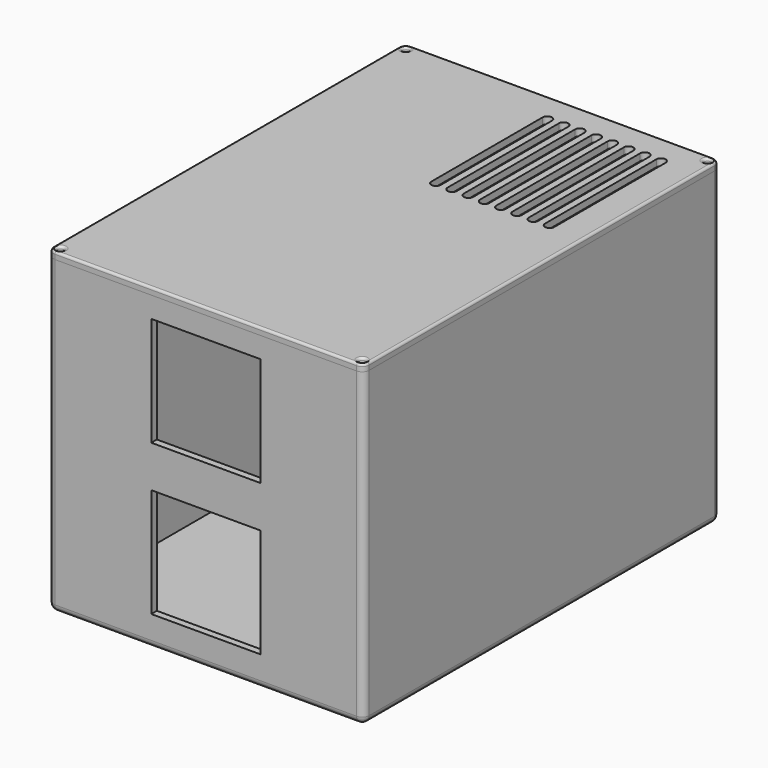
from build123d import *

# Parameters (mm, degrees)
F0_W          = 136
F0_H          = 192
F1_DEPTH      = 4
F2_DEPTH      = 134
F3_W          = 47
F3_H          = 47
F4_DEPTH      = 25
F5_W          = 84
F5_H          = 10
F6_DEPTH      = 20
F8_DEPTH      = 10
F9_W          = 10
F9_H          = 107
F10_DEPTH     = 10
F11_R         = 1.5
F12_DEPTH     = 10
F13_W         = 10
F13_H         = 10
F13_W_2       = 27
F13_H_2       = 68
F13_H_3       = 66
F13_H_4       = 19
F13_R         = 1.6
F14_DEPTH     = 25
F15_R         = 3
F16_R         = 3
F17_R         = 3
F19_W         = 67
F19_H         = 127
F19_W_2       = 47
F19_H_2       = 47
F20_DEPTH     = 10
F21_SIZE      = 1
F23_R         = 1.5
F24_DEPTH     = 3
F25_T1_DEPTH  = 186
F25_T3_DEPTH  = 130
F25_T6_ANGLE  = 90
F25_T8_ANGLE  = 90
F25_T10_ANGLE = 90
F25_T12_ANGLE = 90
F27_DEPTH     = 25
F28_W         = 2.2
F28_H         = 59
F28_H_2       = 5
F29_DEPTH     = 97


# Not quite as in the source:
# - a fillet or chamfer that OpenCascade refuses, or shapes differently, is made with other operations: its cross-section is extruded or revolved along the edge and cut away or added


with BuildPart() as f1:
    # F0 (on Top) → F1 (new body)
    with BuildSketch(Plane.XY):
        Rectangle(F0_W, F0_H)
        with BuildLine():
            ThreePointArc((65, -88), (61.4644660941, -89.4644660941), (60, -93))
            Line((60, -93), (-60, -93))
            ThreePointArc((-60, -93), (-61.4644660941, -89.4644660941), (-65, -88))
            Line((-65, -88), (-65, 88))
            ThreePointArc((-65, 88), (-61.4644660941, 89.4644660941), (-60, 93))
            Line((-60, 93), (60, 93))
            ThreePointArc((60, 93), (61.4644660941, 89.4644660941), (65, 88))
            Line((65, 88), (65, -88))
        make_face(mode=Mode.SUBTRACT)
        with BuildLine():
            Line((-60, -93), (60, -93))
            ThreePointArc((60, -93), (61.4644660941, -89.4644660941), (65, -88))
            Line((65, -88), (65, 88))
            ThreePointArc((65, 88), (61.4644660941, 89.4644660941), (60, 93))
            Line((60, 93), (-60, 93))
            ThreePointArc((-60, 93), (-61.4644660941, 89.4644660941), (-65, 88))
            Line((-65, 88), (-65, -88))
            ThreePointArc((-65, -88), (-61.4644660941, -89.4644660941), (-60, -93))
        make_face()
    extrude(amount=F1_DEPTH)

    # F0 (on Top) → F2 (join)
    with BuildSketch(Plane.XY):
        Rectangle(F0_W, F0_H)
        with BuildLine():
            ThreePointArc((65, -88), (61.4644660941, -89.4644660941), (60, -93))
            Line((60, -93), (-60, -93))
            ThreePointArc((-60, -93), (-61.4644660941, -89.4644660941), (-65, -88))
            Line((-65, -88), (-65, 88))
            ThreePointArc((-65, 88), (-61.4644660941, 89.4644660941), (-60, 93))
            Line((-60, 93), (60, 93))
            ThreePointArc((60, 93), (61.4644660941, 89.4644660941), (65, 88))
            Line((65, 88), (65, -88))
        make_face(mode=Mode.SUBTRACT)
    extrude(amount=F2_DEPTH)

    # F3 (on face) → F4 (cut)
    with BuildSketch(Plane.XZ.offset(96)):
        with Locations((0, 101.5)):
            Rectangle(F3_W, F3_H)
        with Locations((0, 36.5)):
            Rectangle(F3_W, F3_H)
    extrude(amount=-F4_DEPTH, mode=Mode.SUBTRACT)

    # F5 (on face) → F6 (join)
    with BuildSketch(Plane.XY.offset(4)):
        with Locations((-23, 78)):
            Rectangle(F5_W, F5_H)
    extrude(amount=F6_DEPTH)

    # F7 (on face) → F8 (cut)
    with BuildSketch(Plane.XZ.offset(-73)):
        Polygon((-28, 14), (-18, 14), (9, 14), (9, 4), (19, 4), (19, 24), (19, 33.6412377656), (-55, 33.6412377656), (-65, 33.6412377656), (-65, 24), (-65, 14), (-55, 14), align=None)
    extrude(amount=-F8_DEPTH, mode=Mode.SUBTRACT)

    # F9 (on face) → F10 (join)
    with BuildSketch(Plane(origin=(65, 0, 0), x_dir=(0, -1, 0), z_dir=(-1, 0, 0))):
        with Locations((-78, 57.5)):
            Rectangle(F9_W, F9_H)
        with Locations((-14, 57.5)):
            Rectangle(F9_W, F9_H)
    extrude(amount=F10_DEPTH)

    # F11 (on face) → F12 (cut)
    with BuildSketch(Plane.XY.offset(134)):
        with Locations((65, 93)):
            Circle(F11_R)
        with Locations((-65, 93)):
            Circle(F11_R)
        with Locations((65, -93)):
            Circle(F11_R)
        with Locations((-65, -93)):
            Circle(F11_R)
    extrude(amount=-F12_DEPTH, mode=Mode.SUBTRACT)

    # F13 (on face) → F14 (cut)
    with BuildSketch(Plane(origin=(0, 96, 0), x_dir=(-1, 0, 0), z_dir=(0, 1, 0))):
        with Locations((-40, 129)):
            Rectangle(F13_W, F13_H)
        with Locations((41.5, 48)):
            Rectangle(F13_W_2, F13_H_2)
        with Locations((4.5, 48)):
            Rectangle(F13_W_2, F13_H_3)
        with Locations((-24, 26.5)):
            Rectangle(F13_W, F13_H_4)
        with Locations((-24, 14)):
            Circle(F13_R)
        with Locations((-24, 39)):
            Circle(F13_R)
        with Locations((-24, 49)):
            Circle(F13_R)
        with Locations((-24, 61.5)):
            Rectangle(F13_W, F13_H_4)
        with Locations((-24, 74)):
            Circle(F13_R)
    extrude(amount=-F14_DEPTH, mode=Mode.SUBTRACT)

    # F15
    f15_edges = [f1.edges().sort_by_distance(p)[0] for p in [
        (-68, -96, 67),
        (68, -96, 67),
        (68, 96, 67),
        (-68, 96, 67),
    ]]
    fillet(f15_edges, radius=F15_R)

    # F16
    f16_edges = [f1.edges().sort_by_distance(p)[0] for p in [
        (0, -96, 0),
    ]]
    fillet(f16_edges, radius=F16_R)

    # F17
    f17_edges = [f1.edges().sort_by_distance(p)[0] for p in [
        (45, 94.5, 124),
        (35, 94.5, 124),
    ]]
    fillet(f17_edges, radius=F17_R)

    # F28 (on face) → F29 (cut)
    with BuildSketch(Plane.XY.offset(111)):
        with Locations((60, 48.5)):
            Rectangle(F28_W, F28_H)
        with Locations((60, 16.5)):
            Rectangle(F28_W, F28_H_2)
    extrude(amount=-F29_DEPTH, mode=Mode.SUBTRACT)


with BuildPart() as f20:
    # F19 (on offset) → F20 (new body)
    with BuildSketch(Plane(origin=(0, -23, 0), x_dir=(-1, 0, 0), z_dir=(0, 1, 0))):
        with Locations((0, 66.5)):
            Rectangle(F19_W, F19_H)
        with Locations((0, 36.5)):
            Rectangle(F19_W_2, F19_H_2, mode=Mode.SUBTRACT)
        with Locations((0, 101.5)):
            Rectangle(F19_W_2, F19_H_2, mode=Mode.SUBTRACT)
    extrude(amount=F20_DEPTH)

    # F21
    f21_edges = [f20.edges().sort_by_distance(p)[0] for p in [
        (-33.5, -23, 66.5),
        (0, -23, 130),
        (33.5, -23, 66.5),
        (0, -23, 3),
        (23.5, -23, 36.5),
        (0, -23, 60),
        (-23.5, -23, 36.5),
        (0, -23, 13),
        (23.5, -23, 101.5),
        (0, -23, 125),
        (-23.5, -23, 101.5),
        (0, -23, 78),
        (-33.5, -13, 66.5),
        (0, -13, 130),
        (33.5, -13, 66.5),
        (0, -13, 3),
        (23.5, -13, 36.5),
        (0, -13, 60),
        (-23.5, -13, 36.5),
        (0, -13, 13),
        (23.5, -13, 101.5),
        (0, -13, 125),
        (-23.5, -13, 101.5),
        (0, -13, 78),
    ]]
    chamfer(f21_edges, length=F21_SIZE)


with BuildPart() as f24:
    # F23 (on offset) → F24 (new body)
    with BuildSketch(Plane.XY.offset(134)):
        with BuildLine():
            ThreePointArc((65, -96), (67.1213203436, -95.1213203436), (68, -93))
            Line((68, -93), (68, 93))
            ThreePointArc((68, 93), (67.1213203436, 95.1213203436), (65, 96))
            Line((65, 96), (-65, 96))
            ThreePointArc((-65, 96), (-67.1213203436, 95.1213203436), (-68, 93))
            Line((-68, 93), (-68, -93))
            ThreePointArc((-68, -93), (-67.1213203436, -95.1213203436), (-65, -96))
            Line((-65, -96), (65, -96))
        make_face()
        with Locations((-65, -93)):
            Circle(F23_R, mode=Mode.SUBTRACT)
        with Locations((65, -93)):
            Circle(F23_R, mode=Mode.SUBTRACT)
        with Locations((-65, 93)):
            Circle(F23_R, mode=Mode.SUBTRACT)
        with BuildLine():
            Line((-60, 93), (60, 93))
            ThreePointArc((60, 93), (61.4644660941, 89.4644660941), (65, 88))
            Line((65, 88), (65, -88))
            ThreePointArc((65, -88), (61.4644660941, -89.4644660941), (60, -93))
            Line((60, -93), (-60, -93))
            ThreePointArc((-60, -93), (-61.4644660941, -89.4644660941), (-65, -88))
            Line((-65, -88), (-65, 88))
            ThreePointArc((-65, 88), (-61.4644660941, 89.4644660941), (-60, 93))
        make_face(mode=Mode.SUBTRACT)
        with Locations((65, 93)):
            Circle(F23_R, mode=Mode.SUBTRACT)
        with BuildLine():
            ThreePointArc((65, 88), (61.4644660941, 89.4644660941), (60, 93))
            Line((60, 93), (-60, 93))
            ThreePointArc((-60, 93), (-61.4644660941, 89.4644660941), (-65, 88))
            Line((-65, 88), (-65, -88))
            ThreePointArc((-65, -88), (-61.4644660941, -89.4644660941), (-60, -93))
            Line((-60, -93), (60, -93))
            ThreePointArc((60, -93), (61.4644660941, -89.4644660941), (65, -88))
            Line((65, -88), (65, 88))
        make_face()
        with BuildLine():
            Line((64, 87.0839202169), (64, -87.0839202169))
            ThreePointArc((64, -87.0839202169), (60.7573593129, -88.7573593129), (59.0839202169, -92))
            Line((59.0839202169, -92), (-59.0839202169, -92))
            ThreePointArc((-59.0839202169, -92), (-60.7573593129, -88.7573593129), (-64, -87.0839202169))
            Line((-64, -87.0839202169), (-64, 87.0839202169))
            ThreePointArc((-64, 87.0839202169), (-60.7573593129, 88.7573593129), (-59.0839202169, 92))
            Line((-59.0839202169, 92), (59.0839202169, 92))
            ThreePointArc((59.0839202169, 92), (60.7573593129, 88.7573593129), (64, 87.0839202169))
        make_face(mode=Mode.SUBTRACT)
        with BuildLine():
            ThreePointArc((59.0839202169, -92), (60.7573593129, -88.7573593129), (64, -87.0839202169))
            Line((64, -87.0839202169), (64, 87.0839202169))
            ThreePointArc((64, 87.0839202169), (60.7573593129, 88.7573593129), (59.0839202169, 92))
            Line((59.0839202169, 92), (-59.0839202169, 92))
            ThreePointArc((-59.0839202169, 92), (-60.7573593129, 88.7573593129), (-64, 87.0839202169))
            Line((-64, 87.0839202169), (-64, -87.0839202169))
            ThreePointArc((-64, -87.0839202169), (-60.7573593129, -88.7573593129), (-59.0839202169, -92))
            Line((-59.0839202169, -92), (59.0839202169, -92))
        make_face()
    extrude(amount=F24_DEPTH)

    # F25: fillet of radius 1 on 12 edges, made by hand

    # F25_s2 → F25_t1 (cut)
    with BuildSketch(Plane.XZ.offset(-93)):
        with BuildLine():
            ThreePointArc((68, 136), (67.7071067812, 136.7071067812), (67, 137))
            Line((67, 137), (68, 137))
            Line((68, 137), (68, 136))
        make_face()
        with BuildLine():
            ThreePointArc((-68, 136), (-67.7071067812, 136.7071067812), (-67, 137))
            Line((-67, 137), (-68, 137))
            Line((-68, 137), (-68, 136))
        make_face()
    extrude(amount=F25_T1_DEPTH, mode=Mode.SUBTRACT)

    # F25_s4 → F25_t3 (cut)
    with BuildSketch(Plane.YZ.offset(-65)):
        with BuildLine():
            ThreePointArc((96, 136), (95.7071067812, 136.7071067812), (95, 137))
            Line((95, 137), (96, 137))
            Line((96, 137), (96, 136))
        make_face()
        with BuildLine():
            ThreePointArc((-96, 136), (-95.7071067812, 136.7071067812), (-95, 137))
            Line((-95, 137), (-96, 137))
            Line((-96, 137), (-96, 136))
        make_face()
    extrude(amount=F25_T3_DEPTH, mode=Mode.SUBTRACT)

    # F25_s5 → F25_t6 (revolve, cut)
    with BuildSketch(Plane.YZ.offset(65)):
        with BuildLine():
            ThreePointArc((-96, 136), (-95.7071067812, 136.7071067812), (-95, 137))
            Line((-95, 137), (-96, 137))
            Line((-96, 137), (-96, 136))
        make_face()
    revolve(axis=Axis((65, -93, 137), (0, 0, 1)), revolution_arc=F25_T6_ANGLE, mode=Mode.SUBTRACT)

    # F25_s7 → F25_t8 (revolve, cut)
    with BuildSketch(Plane.XZ.offset(-93)):
        with BuildLine():
            ThreePointArc((68, 136), (67.7071067812, 136.7071067812), (67, 137))
            Line((67, 137), (68, 137))
            Line((68, 137), (68, 136))
        make_face()
    revolve(axis=Axis((65, 93, 137), (0, 0, 1)), revolution_arc=F25_T8_ANGLE, mode=Mode.SUBTRACT)

    # F25_s9 → F25_t10 (revolve, cut)
    with BuildSketch(Plane.YZ.offset(-65)):
        with BuildLine():
            ThreePointArc((96, 136), (95.7071067812, 136.7071067812), (95, 137))
            Line((95, 137), (96, 137))
            Line((96, 137), (96, 136))
        make_face()
    revolve(axis=Axis((-65, 93, 137), (0, 0, 1)), revolution_arc=F25_T10_ANGLE, mode=Mode.SUBTRACT)

    # F25_s11 → F25_t12 (revolve, cut)
    with BuildSketch(Plane.XZ.offset(93)):
        with BuildLine():
            ThreePointArc((-68, 136), (-67.7071067812, 136.7071067812), (-67, 137))
            Line((-67, 137), (-68, 137))
            Line((-68, 137), (-68, 136))
        make_face()
    revolve(axis=Axis((-65, -93, 137), (0, 0, 1)), revolution_arc=F25_T12_ANGLE, mode=Mode.SUBTRACT)

    # F25_s13 → F25_t14 (revolve, cut)
    with BuildSketch(Plane.XZ.offset(93)):
        with BuildLine():
            ThreePointArc((-63.5, 136), (-63.2071067812, 136.7071067812), (-62.5, 137))
            Line((-62.5, 137), (-63.5, 137))
            Line((-63.5, 137), (-63.5, 136))
        make_face()
    revolve(axis=Axis((-65, -93, 137), (0, 0, 1)), mode=Mode.SUBTRACT)

    # F25_s15 → F25_t16 (revolve, cut)
    with BuildSketch(Plane.XZ.offset(93)):
        with BuildLine():
            ThreePointArc((66.5, 136), (66.7928932188, 136.7071067812), (67.5, 137))
            Line((67.5, 137), (66.5, 137))
            Line((66.5, 137), (66.5, 136))
        make_face()
    revolve(axis=Axis((65, -93, 137), (0, 0, 1)), mode=Mode.SUBTRACT)

    # F25_s17 → F25_t18 (revolve, cut)
    with BuildSketch(Plane.XZ.offset(-93)):
        with BuildLine():
            ThreePointArc((-63.5, 136), (-63.2071067812, 136.7071067812), (-62.5, 137))
            Line((-62.5, 137), (-63.5, 137))
            Line((-63.5, 137), (-63.5, 136))
        make_face()
    revolve(axis=Axis((-65, 93, 137), (0, 0, 1)), mode=Mode.SUBTRACT)

    # F25_s19 → F25_t20 (revolve, cut)
    with BuildSketch(Plane.XZ.offset(-93)):
        with BuildLine():
            ThreePointArc((66.5, 136), (66.7928932188, 136.7071067812), (67.5, 137))
            Line((67.5, 137), (66.5, 137))
            Line((66.5, 137), (66.5, 136))
        make_face()
    revolve(axis=Axis((65, 93, 137), (0, 0, 1)), mode=Mode.SUBTRACT)

    # F26 (on face) → F27 (cut)
    with BuildSketch(Plane.XY.offset(137)):
        with BuildLine():
            ThreePointArc((6, 83), (4, 85), (2, 83))
            Line((2, 83), (2, 23))
            ThreePointArc((2, 23), (4, 21), (6, 23))
            Line((6, 23), (6, 83))
        make_face()
        with BuildLine():
            Line((13, 23), (13, 83))
            ThreePointArc((13, 83), (11, 85), (9, 83))
            Line((9, 83), (9, 23))
            ThreePointArc((9, 23), (11, 21), (13, 23))
        make_face()
        with BuildLine():
            Line((20, 23), (20, 83))
            ThreePointArc((20, 83), (18, 85), (16, 83))
            Line((16, 83), (16, 23))
            ThreePointArc((16, 23), (18, 21), (20, 23))
        make_face()
        with BuildLine():
            Line((27, 23), (27, 83))
            ThreePointArc((27, 83), (25, 85), (23, 83))
            Line((23, 83), (23, 23))
            ThreePointArc((23, 23), (25, 21), (27, 23))
        make_face()
        with BuildLine():
            Line((34, 23), (34, 83))
            ThreePointArc((34, 83), (32, 85), (30, 83))
            Line((30, 83), (30, 23))
            ThreePointArc((30, 23), (32, 21), (34, 23))
        make_face()
        with BuildLine():
            Line((41, 23), (41, 83))
            ThreePointArc((41, 83), (39, 85), (37, 83))
            Line((37, 83), (37, 23))
            ThreePointArc((37, 23), (39, 21), (41, 23))
        make_face()
        with BuildLine():
            Line((48, 23), (48, 83))
            ThreePointArc((48, 83), (46, 85), (44, 83))
            Line((44, 83), (44, 23))
            ThreePointArc((44, 23), (46, 21), (48, 23))
        make_face()
        with BuildLine():
            Line((55, 23), (55, 83))
            ThreePointArc((55, 83), (53, 85), (51, 83))
            Line((51, 83), (51, 23))
            ThreePointArc((51, 23), (53, 21), (55, 23))
        make_face()
    extrude(amount=-F27_DEPTH, mode=Mode.SUBTRACT)


solid = Compound([f1.part, f20.part, f24.part])
